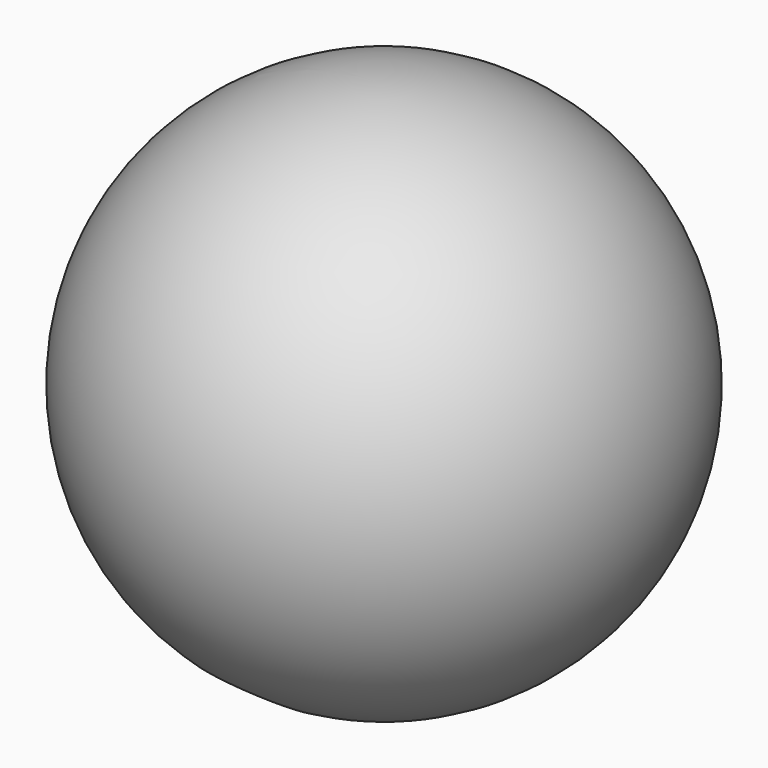
from build123d import *

# Parameters (mm, degrees)
F4_R         = 3.175
F5_DEPTH     = 38.1
F6_TEXT_SIZE = 3.6323591808
F7_DEPTH     = 31.75
F9_ANGLE     = -120


# Not quite as in the source:
# - Text() gives the source's letters only with a copy of the font that has no kerning and outlines rounded to 1/6400 em; it was checked with that copy


with BuildPart() as f2:
    # F1 (on Front) → F2 (revolve)
    with BuildSketch(Plane.XZ):
        with BuildLine():
            Line((0, -15.875), (0, 15.875))
            ThreePointArc((0, 15.875), (-15.875, 0), (0, -15.875))
        make_face()
    revolve(axis=Axis((0, 0, 0), (0, 0, 1)))

    # F6 (on face) → F7 (cut)
    with BuildSketch(Plane(origin=(0, 44.45, 0), x_dir=(-1, 0, 0), z_dir=(0, 1, 0))):
        with Locations((-4.653544187, 4.386571236)):
            Text('104.45', F6_TEXT_SIZE, font='Open Sans', text_align=(TextAlign.LEFT, TextAlign.BOTTOM))
    extrude(amount=-F7_DEPTH, mode=Mode.SUBTRACT)


with BuildPart() as f5:
    # F4 (on offset) → F5 (new body)
    with BuildSketch(Plane.XZ.offset(-6.35)):
        with Locations((-1.5955890995, 0)):
            Circle(F4_R)
    extrude(amount=-F5_DEPTH)


with BuildPart() as f9_1:
    # F9: copy of F5
    add(f5.part.rotate(Axis((19.8181457818, 0, 0), (1, 0, 0)), F9_ANGLE))


with BuildPart() as f2_1:
    add(f2.part)

    # F10: cut F9_1, F5
    add(f9_1.part, mode=Mode.SUBTRACT)
    add(f5.part, mode=Mode.SUBTRACT)


solid = f2_1.part
